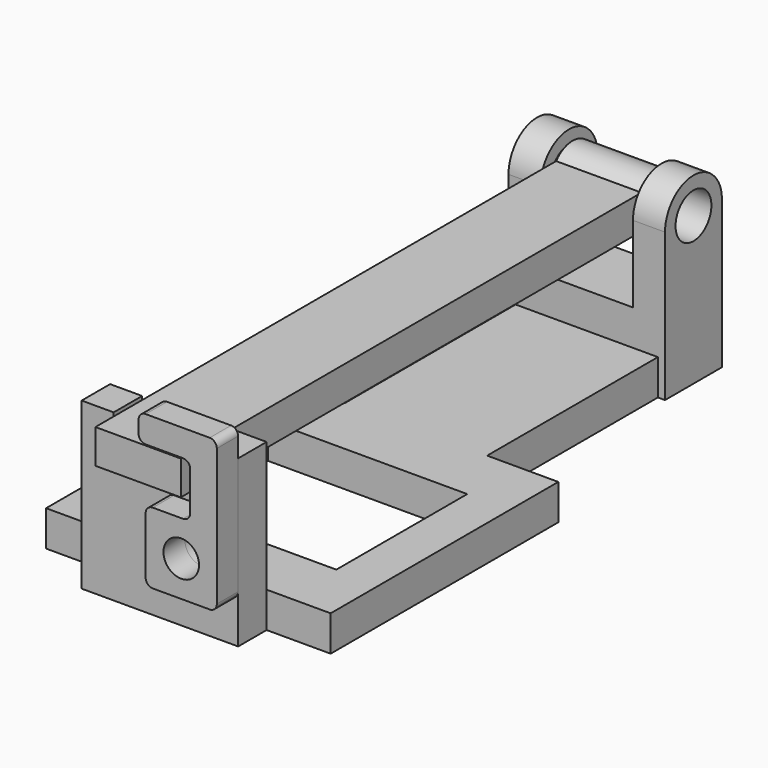
from build123d import *

# Parameters (mm, degrees)
F0_W          = 35.56
F0_H          = 29.21
F1_DEPTH      = 6.35
F2_R          = 4.0005
F2_W          = 6.35
F2_H          = 29.5656
F3_DEPTH      = 13.97
F3_DEPTH_BACK = 13.97
F4_W          = 16.51
F4_H          = 11.7008156112
F4_H_2        = 13.6991843888
F5_DEPTH      = 12.701
F6_R          = 2.5
F7_DEPTH      = 7.62
F7_DEPTH_BACK = 7.62
F8_W          = 16.51
F8_H          = 6.35
F9_DEPTH      = 106.3635
F10_R         = 3.175
F11_DEPTH     = 4.7625
F12_DEPTH     = 6.35


with BuildPart() as f1:
    # F0 (on Top) → F1 (new body)
    with BuildSketch(Plane.XY):
        Polygon((-12.7, 25.4), (-25.4, 25.4), (-25.4, -25.4), (25.4, -25.4), (25.4, 25.4), (12.7, 25.4), (12.7, 63.5), (-12.7, 63.5), align=None)
        Rectangle(F0_W, F0_H, mode=Mode.SUBTRACT)
    extrude(amount=F1_DEPTH)

    # F2 (on Right) → F3 (join, two sides)
    with BuildSketch(Plane.YZ) as f3_sk:
        with BuildLine():
            Line((76.2, 0), (76.2, 26.3991843888))
            ThreePointArc((76.2, 26.3991843888), (69.85, 32.7491843888), (63.5, 26.3991843888))
            Line((63.5, 26.3991843888), (63.5, 0))
            Line((63.5, 0), (76.2, 0))
        make_face()
        with Locations((69.85, 26.3991843888)):
            Circle(F2_R, mode=Mode.SUBTRACT)
        with Locations((-28.575, 14.7828)):
            Rectangle(F2_W, F2_H)
    extrude(amount=F3_DEPTH)
    extrude(f3_sk.sketch, amount=-F3_DEPTH_BACK)

    # F4 (on face) → F5 (cut, through all)
    with BuildSketch(Plane.XZ.offset(-63.5)):
        with Locations((0, 32.2495921944)):
            Rectangle(F4_W, F4_H)
        with Locations((0, 19.5495921944)):
            Rectangle(F4_W, F4_H_2)
    extrude(amount=-F5_DEPTH, mode=Mode.SUBTRACT)

    # F8 (on face) → F9 (cut, through all)
    with BuildSketch(Plane.XZ.offset(31.75)):
        with Locations((0, 26.3906)):
            Rectangle(F8_W, F8_H)
    extrude(amount=-F9_DEPTH, mode=Mode.SUBTRACT)

    # F10 (on face) → F12 (cut, through all)
    with BuildSketch(Plane.XZ.offset(31.75)):
        with Locations((7.62, 13.6906)):
            Circle(F10_R)
    extrude(amount=-F12_DEPTH, mode=Mode.SUBTRACT)


with BuildPart() as f7:
    # F6 (on Right) → F7 (new body, two sides)
    with BuildSketch(Plane.YZ) as f7_sk:
        with BuildLine():
            Line((-36.6158854962, 23.3511843888), (66.1906144983, 23.3511843888))
            ThreePointArc((66.1906144983, 23.3511843888), (74.6125, 26.3991843888), (66.1906144983, 29.4471843888))
            Line((66.1906144983, 29.4471843888), (-36.6158855017, 29.4471843888))
            Line((-36.6158855017, 29.4471843888), (-36.6158854962, 23.3511843888))
        make_face()
        with Locations((69.85, 26.3991843888)):
            Circle(F6_R, mode=Mode.SUBTRACT)
    extrude(amount=F7_DEPTH)
    extrude(f7_sk.sketch, amount=-F7_DEPTH_BACK)


with BuildPart() as f11:
    # F10 (on face) → F11 (new body)
    with BuildSketch(Plane.XZ.offset(31.75)):
        with BuildLine():
            Line((8.255, 29.5656), (8.255, 29.5252722124))
            ThreePointArc((8.255, 29.5252722124), (8.9415231571, 29.0733129933), (9.2075, 28.2956))
            Line((9.2075, 28.2956), (9.2075, 21.3106))
            ThreePointArc((9.2075, 21.3106), (8.8355256121, 20.4125743879), (7.9375, 20.0406))
            Line((7.9375, 20.0406), (2.54, 20.0406))
            ThreePointArc((2.54, 20.0406), (1.6419743879, 19.6686256121), (1.27, 18.7706))
            Line((1.27, 18.7706), (1.27, 8.6106))
            ThreePointArc((1.27, 8.6106), (1.6419743879, 7.7125743879), (2.54, 7.3406))
            Line((2.54, 7.3406), (12.7, 7.3406))
            ThreePointArc((12.7, 7.3406), (13.5980256121, 7.7125743879), (13.97, 8.6106))
            Line((13.97, 8.6106), (13.97, 29.5656))
            Line((13.97, 29.5656), (8.255, 29.5656))
        make_face()
        with Locations((7.62, 13.6906)):
            Circle(F10_R, mode=Mode.SUBTRACT)
        with BuildLine():
            Line((0, 33.0581), (0, 30.8356))
            ThreePointArc((0, 30.8356), (0.3719743879, 29.9375743879), (1.27, 29.5656))
            Line((1.27, 29.5656), (7.9375, 29.5656))
            ThreePointArc((7.9375, 29.5656), (8.0975254515, 29.5554777143), (8.255, 29.5252722124))
            Line((8.255, 29.5252722124), (8.255, 29.5656))
            Line((8.255, 29.5656), (13.97, 29.5656))
            Line((13.97, 29.5656), (13.97, 33.0581))
            ThreePointArc((13.97, 33.0581), (13.5980256121, 33.9561256121), (12.7, 34.3281))
            Line((12.7, 34.3281), (1.27, 34.3281))
            ThreePointArc((1.27, 34.3281), (0.3719743879, 33.9561256121), (0, 33.0581))
        make_face()
    extrude(amount=F11_DEPTH)


solid = Compound([f1.part, f7.part, f11.part])
